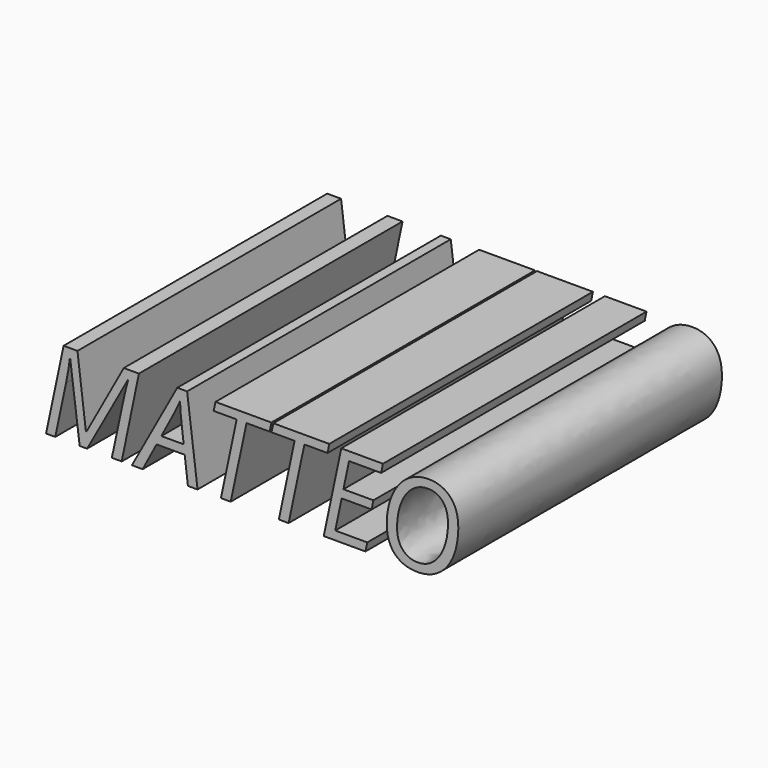
from build123d import *

# Parameters (mm, degrees)
F0_TEXT_SIZE = 8.9571759519
F1_DEPTH     = 25.4


# Not quite as in the source:
# - Text() gives the source's letters only with a copy of the font that has no kerning and outlines rounded to 1/6400 em; it was checked with that copy


with BuildPart() as f1:
    # F0 (on Front) → F1 (new body)
    with BuildSketch(Plane.XZ):
        with Locations((-60.3601895273, 29.1220284998)):
            Text('MATTEO', F0_TEXT_SIZE, font='Open Sans', font_style=FontStyle.ITALIC, text_align=(TextAlign.LEFT, TextAlign.BOTTOM))
    extrude(amount=F1_DEPTH)


solid = f1.part
